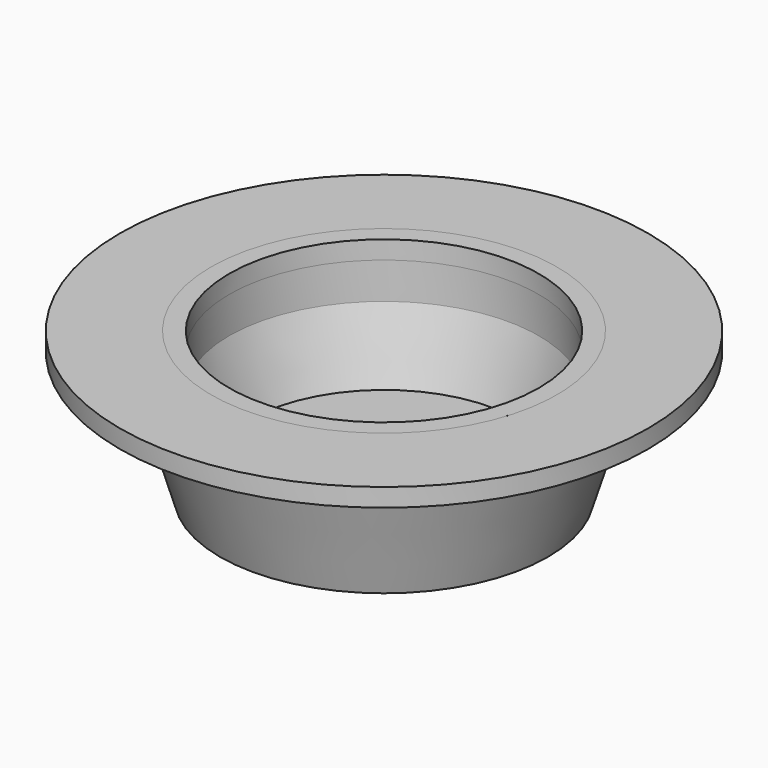
from build123d import *


# Not quite as in the source:
# - ends of sketch curves that miss each other by under 0.0002 mm in the source are joined


with BuildPart() as f1:
    # F0 (on Front) → F1 (revolve)
    with BuildSketch(Plane.XZ):
        Polygon((-7, 0), (0, 0), (0, 1.3), (-7.3899972171, 1.3), align=None)
        Polygon((-9, 0), (-7, 0), (-7.3899972171, 1.3), (-9, 1.3), align=None)
        Polygon((-10.4999892964, 4.9999928643), (-9, 0), (-9, 1.3), (-7.3899972171, 1.3), (-8.4999892965, 5), (-9.4999892964, 4.9999964322), align=None)
        Polygon((-9.4999892964, 4.9999964322), (-8.4999892965, 5), (-8.4999964322, 7), (-9.4999964321, 6.9999964322), align=None)
        Polygon((-9.4999964321, 6.9999964322), (-8.4999964322, 7), (-8.5, 8), (-9.4999964321, 8), align=None)
        Polygon((-14.5, 7), (-9.4999964321, 7), (-9.4999964321, 7.9999964322), (-14.5, 8), align=None)
    revolve(axis=Axis((0, 0, 0.65), (0, 0, 1)))


solid = f1.part
